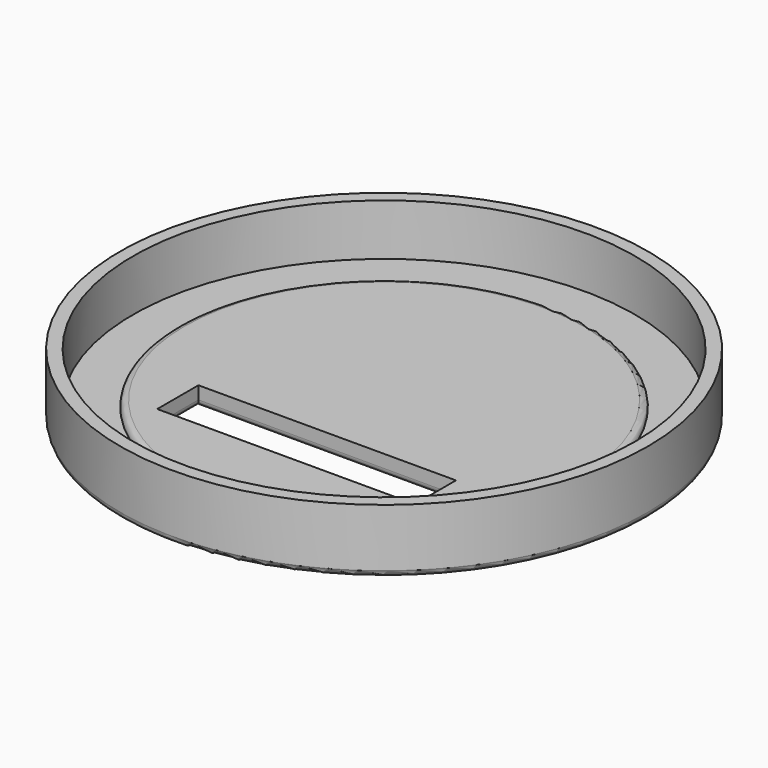
from build123d import *

# Parameters (mm, degrees)
F0_R           = 41
F1_DEPTH       = 10
F2_R           = 39
F2_R_2         = 32
F3_DEPTH       = 8
F4_DEPTH       = 7
F5_TEXT_SIZE   = 13.198045609
F5_TEXT_SIZE_2 = 13.1736111111
F6_DEPTH       = 0.4
F7_W           = 40
F7_H           = 8
F8_DEPTH       = 25
F9_R           = 0.99999
F10_SCALE      = 1.02


# Not quite as in the source:
# - a fillet or chamfer is up to 0.001 mm smaller than in the source, because OpenCascade refuses the exact size
# - Text() gives the source's letters only with a copy of the font that has no kerning and outlines rounded to 1/6400 em; it was checked with that copy


with BuildPart() as f1:
    # F0 (on Top) → F1 (new body)
    with BuildSketch(Plane.XY):
        Circle(F0_R)
    extrude(amount=F1_DEPTH)

    # F2 (on face) → F3 (cut)
    with BuildSketch(Plane.XY.offset(10)):
        Circle(F2_R)
        Circle(F2_R_2, mode=Mode.SUBTRACT)
    extrude(amount=-F3_DEPTH, mode=Mode.SUBTRACT)

    # F4 (cut): a face of the model
    f4_faces = [f1.faces().sort_by_distance(p)[0] for p in [
        (0, 0, 10),
    ]]
    extrude(f4_faces, amount=-F4_DEPTH, mode=Mode.SUBTRACT)

    # F5 (on face) → F6 (cut)
    with BuildSketch(Plane(origin=(0, 0, 0), x_dir=(1, 0, 0), z_dir=(0, 0, -1))):
        with Locations((-29.6213636137, -4.7512964192)):
            Text('HONESTY', F5_TEXT_SIZE, font='Open Sans', text_align=(TextAlign.LEFT, TextAlign.BOTTOM))
        with Locations((-10.6281563712, -18.5694172978)):
            Text('JAR', F5_TEXT_SIZE_2, font='Open Sans', text_align=(TextAlign.LEFT, TextAlign.BOTTOM))
    extrude(amount=-F6_DEPTH, mode=Mode.SUBTRACT)

    # F7 (on face) → F8 (cut)
    with BuildSketch(Plane(origin=(0, 0, 0), x_dir=(1, 0, 0), z_dir=(0, 0, -1))):
        with Locations((-0.0077676401, 15.0385912525)):
            Rectangle(F7_W, F7_H)
    extrude(amount=-F8_DEPTH, mode=Mode.SUBTRACT)

    # F9 (radius 1 in the source; OpenCascade refuses exactly that, so slightly less here)
    f9_edges = [f1.edges().sort_by_distance(p)[0] for p in [
        (-41, 0, 0),
        (-0.007768, -19.038591, 0),
        (-20.007768, -15.038591, 0),
        (-0.007768, -11.038591, 0),
        (19.992232, -15.038591, 0),
        (-32, 0, 3),
    ]]
    fillet(f9_edges, radius=F9_R)


with BuildPart() as f1_1:
    # F10: moved
    add(f1.part.scale(F10_SCALE))


solid = f1_1.part
